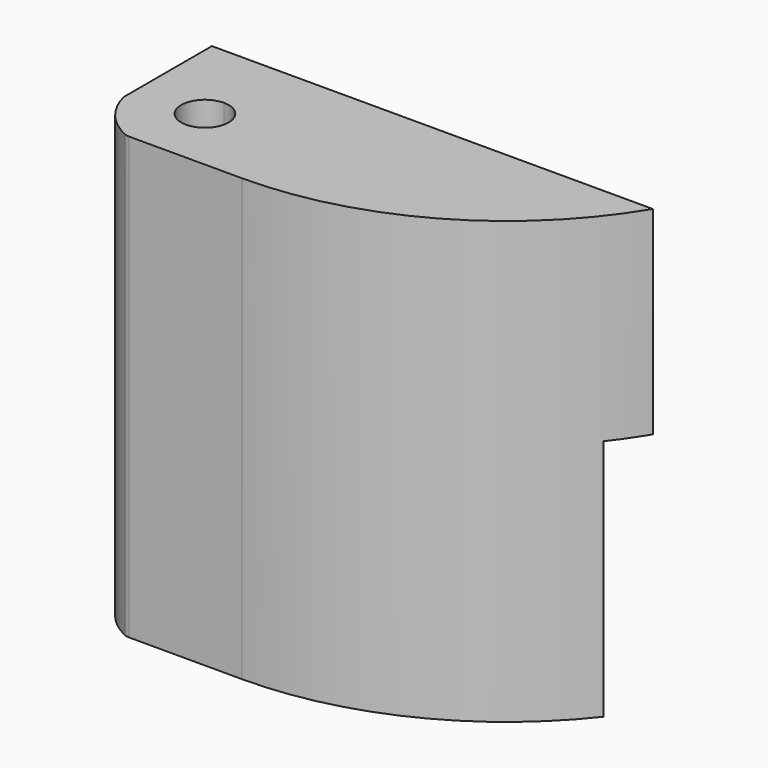
from build123d import *

# Parameters (mm, degrees)
F0_W        = 6.1
F0_H        = 3
F0_W_2      = 27.8
F1_DEPTH    = 40
F2_R        = 1
F3_T1_DEPTH = 168.4279953904
F4_DEPTH    = 22


# Not quite as in the source:
# - a fillet or chamfer that OpenCascade refuses, or shapes differently, is made with other operations: its cross-section is extruded or revolved along the edge and cut away or added


with BuildPart() as f1:
    # F0 (on Top) → F1 (new body)
    with BuildSketch(Plane.XY):
        with Locations((3.05, 6.91)):
            Rectangle(F0_W, F0_H)
        with Locations((-3.05, 6.91)):
            Rectangle(F0_W, F0_H)
        with BuildLine():
            Line((6.1, -1.59), (6.1, 5.41))
            Line((6.1, 5.41), (0, 5.41))
            Line((0, 5.41), (0, 2.15))
            ThreePointArc((0, 2.15), (1.5202795796, 1.5202795796), (2.15, 0))
            ThreePointArc((2.15, 0), (1.5202795796, -1.5202795796), (0, -2.15))
            Line((0, -2.15), (0, -6.09))
            Line((0, -6.09), (2.25, -6.09))
            ThreePointArc((2.25, -6.09), (4.7073896383, -4.2954889128), (6.1, -1.59))
        make_face()
        with Locations((20, 6.91)):
            Rectangle(F0_W_2, F0_H)
        with BuildLine():
            Line((33.9, 5.41), (6.1, 5.41))
            Line((6.1, 5.41), (6.1, -1.59))
            ThreePointArc((6.1, -1.59), (4.7073896383, -4.2954889128), (2.25, -6.09))
            Line((2.25, -6.09), (33.9, -6.09))
            Line((33.9, -6.09), (33.9, 5.41))
        make_face()
        with BuildLine():
            Line((0, 2.15), (0, 5.41))
            Line((0, 5.41), (-6.1, 5.41))
            Line((-6.1, 5.41), (-6.1, -1.59))
            ThreePointArc((-6.1, -1.59), (-4.7073896383, -4.2954889128), (-2.25, -6.09))
            Line((-2.25, -6.09), (0, -6.09))
            Line((0, -6.09), (0, -2.15))
            ThreePointArc((0, -2.15), (-2.15, 0), (0, 2.15))
        make_face()
    extrude(amount=F1_DEPTH)

    # F2
    f2_edges = [f1.edges().sort_by_distance(p)[0] for p in [
        (-2.25, -6.09, 20),
    ]]
    fillet(f2_edges, radius=F2_R)

    # F3: fillet of radius 30 on 1 edges, made by hand

    # F3_s2 → F3_t1 (cut)
    with BuildSketch(Plane.XY.offset(-64.2139976952)):
        with BuildLine():
            ThreePointArc((8.2144009219, -6.09), (22.9622821257, -2.2147009552), (33.9, 8.41))
            Line((33.9, 8.41), (33.9, -6.09))
            Line((33.9, -6.09), (8.2144009219, -6.09))
        make_face()
    extrude(amount=F3_T1_DEPTH, mode=Mode.SUBTRACT)

    # F0 (on Top) → F4 (cut)
    with BuildSketch(Plane.XY):
        with Locations((-3.05, 6.91)):
            Rectangle(F0_W, F0_H)
        with Locations((3.05, 6.91)):
            Rectangle(F0_W, F0_H)
        with Locations((20, 6.91)):
            Rectangle(F0_W_2, F0_H)
    extrude(amount=F4_DEPTH, mode=Mode.SUBTRACT)


solid = f1.part
